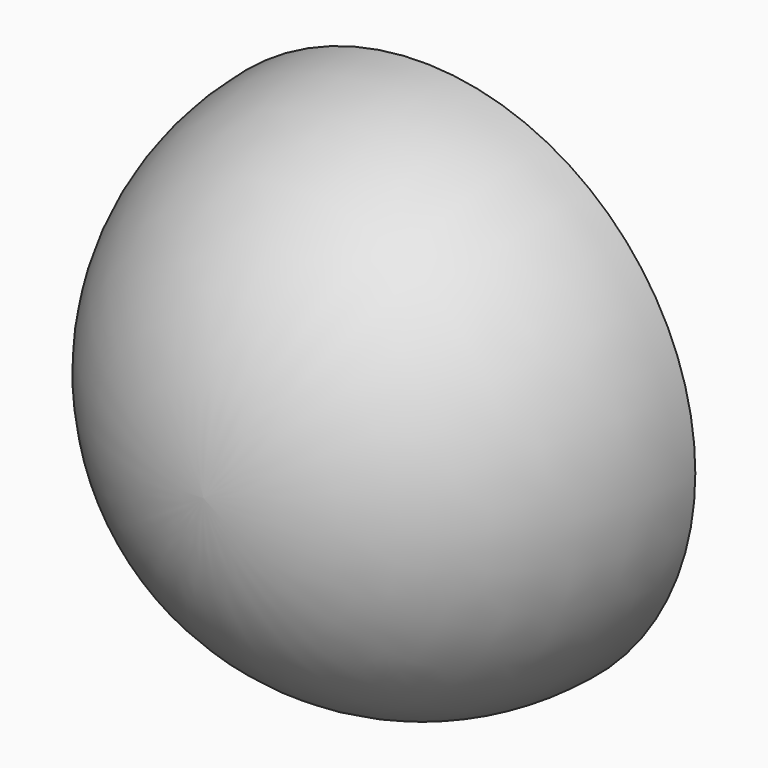
from build123d import *

# Parameters (mm, degrees)
F1_DEPTH = 8
F0_R     = 12.5
F2_R     = 12.5
F3_DEPTH = 12.5
F4_R     = 12.49999
F7_DEPTH = 8


# Not quite as in the source:
# - a fillet or chamfer is up to 0.001 mm smaller than in the source, because OpenCascade refuses the exact size


with BuildPart() as f1:
    # F0 (on Front) → F1 (new body)
    with BuildSketch(Plane.XZ):
        with BuildLine():
            ThreePointArc((0.1338848412, 2.0937357457), (0.1198892217, 2.2981641713), (0.0781635329, 2.4987777937))
            ThreePointArc((0.0781635329, 2.4987777937), (-1.3661151588, 2.0937357457), (-2.3185923934, 0.9349488293))
            ThreePointArc((-2.3185923934, 0.9349488293), (-0.7253015556, 0.7375064414), (0.1338848412, 2.0937357457))
        make_face()
    extrude(amount=F1_DEPTH)


with BuildPart() as f1b:
    # F0 (on Front) → F1, piece 2 (new body)
    with BuildSketch(Plane.XZ):
        Circle(F0_R)
        with BuildLine():
            ThreePointArc((0.0781635329, 2.4987777937), (1.7951892424, 1.7399125219), (2.5, 0))
            ThreePointArc((2.5, 0), (-0.4761927218, -2.4542291033), (-2.3185923934, 0.9349488293))
            ThreePointArc((-2.3185923934, 0.9349488293), (-2.1857842541, 3.3499771931), (0.0781635329, 2.4987777937))
        make_face(mode=Mode.SUBTRACT)
    extrude(amount=F1_DEPTH)


with BuildPart() as f3:
    # F2 (on Front) → F3 (new body)
    with BuildSketch(Plane.XZ):
        Circle(F2_R)
    extrude(amount=F3_DEPTH)

    # F4 (radius 12.5 in the source; OpenCascade refuses exactly that, so slightly less here)
    f4_edges = [f3.edges().sort_by_distance(p)[0] for p in [
        (-12.5, -12.5, 0),
    ]]
    fillet(f4_edges, radius=F4_R)

    # F6 (on Front) → F7 (cut)
    with BuildSketch(Plane.XZ):
        with BuildLine():
            ThreePointArc((2.05, -1.4309088021), (2.3848480035, -0.75), (2.5, 0))
            ThreePointArc((2.5, 0), (2.3848480035, 0.75), (2.05, 1.4309088021))
            ThreePointArc((2.05, 1.4309088021), (1, 0), (2.05, -1.4309088021))
        make_face()
        with BuildLine():
            ThreePointArc((2.05, 1.4309088021), (2.3848480035, 0.75), (2.5, 0))
            ThreePointArc((2.5, 0), (2.3848480035, -0.75), (2.05, -1.4309088021))
            ThreePointArc((2.05, -1.4309088021), (3.3874119675, -1.2093386622), (4, 0))
            ThreePointArc((4, 0), (3.3874119675, 1.2093386622), (2.05, 1.4309088021))
        make_face()
        with BuildLine():
            ThreePointArc((2.05, -1.4309088021), (1, 0), (2.05, 1.4309088021))
            ThreePointArc((2.05, 1.4309088021), (-2.5, 0), (2.05, -1.4309088021))
        make_face()
    extrude(amount=F7_DEPTH, mode=Mode.SUBTRACT)


solid = f3.part
